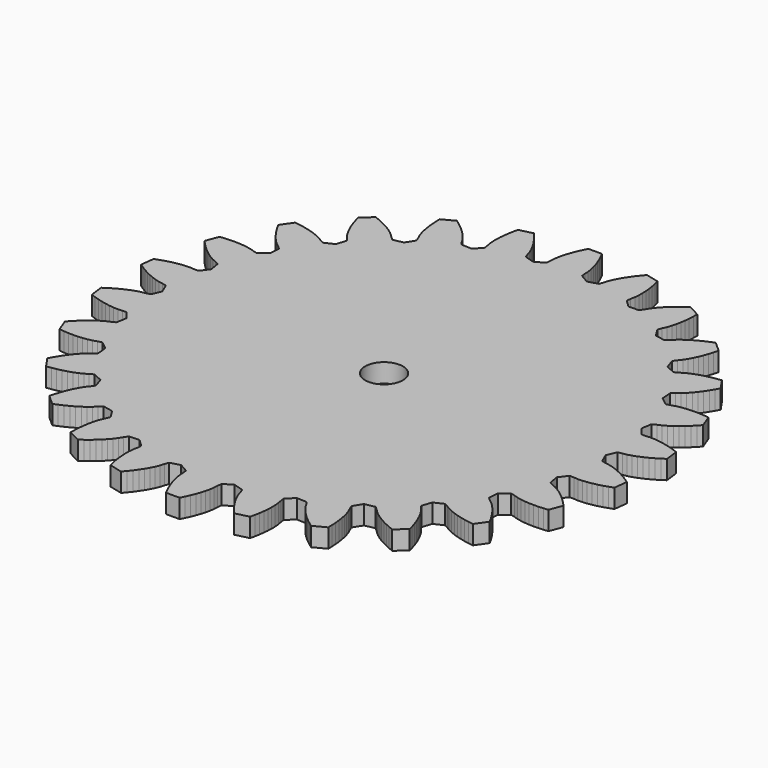
from build123d import *

# Parameters (mm, degrees)
F0_R     = 25.4
F1_DEPTH = 25.4


# Not quite as in the source:
# - ends of sketch curves that miss each other by under 0.0002 mm in the source are joined


with BuildPart() as f1:
    # F0 (on Top) → F1 (new body)
    with BuildSketch(Plane.XY):
        Polygon((93.9964592, 342.9519176), (76.148057, 347.3511722), (71.9280248, 342.4118374), (67.9735496, 337.3908416), (64.2982458, 332.291309), (60.9200458, 327.1156526), (57.8641464, 321.8650154), (55.1692572, 316.5382544), (52.9062696, 311.128791), (51.253517, 305.6119872), (49.2553752, 300.1503776), (35.9741724, 296.2739566), (24.0065814, 303.2161576), (23.3735372, 308.9972484), (23.0890826, 314.7492562), (22.1864174, 320.5430978), (20.8446116, 326.3600026), (19.1340994, 332.1894042), (17.0926506, 338.0231238), (14.744573, 343.854024), (12.1066052, 349.6754754), (9.1912948, 355.4812042), (-9.1912948, 355.4812042), (-12.1066052, 349.6754754), (-14.744573, 343.854024), (-17.0926506, 338.0231238), (-19.1340994, 332.1894042), (-20.8446116, 326.3600026), (-22.1864174, 320.5430978), (-23.0890826, 314.7492562), (-23.3735372, 308.9972484), (-24.0065814, 303.2161576), (-35.9741724, 296.2739566), (-49.2553752, 300.1503776), (-51.253517, 305.6119872), (-52.9062696, 311.128791), (-55.1692572, 316.5382544), (-57.8641464, 321.8650154), (-60.9200458, 327.1156526), (-64.2982458, 332.291309), (-67.9735496, 337.3908416), (-71.9280248, 342.4118374), (-76.1480062, 347.3511722), (-93.9964084, 342.951943), (-95.4376298, 336.6172592), (-96.6057758, 330.3336294), (-97.4902038, 324.1102484), (-98.0762072, 317.9574794), (-98.3419674, 311.888124), (-98.2527118, 305.9191494), (-97.7425782, 300.077632), (-96.6422248, 294.4246842), (-95.8733668, 288.660078), (-105.8318178, 279.0556014), (-119.6548026, 279.6409698), (-122.9019386, 284.4656998), (-125.826901, 289.4266754), (-129.3187152, 294.1373594), (-133.210046, 298.6644014), (-137.4337104, 303.0311694), (-141.9523704, 307.2479504), (-146.741261, 311.3197482), (-151.7824498, 315.2484932), (-157.0618652, 319.0343632), (-173.3388202, 310.4915558), (-173.222158, 303.9960392), (-172.852588, 297.615483), (-172.2219568, 291.3612664), (-171.3185042, 285.2470546), (-170.1240438, 279.2904498), (-168.6089084, 273.5162678), (-166.7156432, 267.9665964), (-164.2944136, 262.7412322), (-162.168332, 257.328162), (-169.5389294, 245.619524), (-183.1003196, 242.8798546), (-187.4077278, 246.787289), (-191.4349232, 250.9040956), (-195.952618, 254.6422644), (-200.8142796, 258.1065196), (-205.9602434, 261.3355708), (-211.3567528, 264.348468), (-216.9809224, 267.1558792), (-222.8158104, 269.7640274), (-228.8478532, 272.1764432), (-242.6074142, 259.9865514), (-240.9396502, 253.7076968), (-239.0538526, 247.600978), (-236.9448144, 241.6793998), (-234.6043822, 235.9590912), (-232.0191448, 230.461439), (-229.166166, 225.2176344), (-225.999802, 220.2823128), (-222.3984122, 215.78824), (-219.038678, 211.041234), (-223.3930254, 197.9089514), (-235.9047098, 192.003426), (-241.0220478, 194.7664888), (-245.917466, 197.7999092), (-251.1984816, 200.3482912), (-256.7479244, 202.5484138), (-262.5171026, 204.4521438), (-268.4778222, 206.0859988), (-274.610449, 207.4658792), (-280.8999462, 208.6018434), (-287.3340456, 209.5006224), (-297.776519, 194.3720522), (-294.654605, 188.6747814), (-291.3621808, 183.1968142), (-287.897316, 177.9520444), (-284.2559212, 172.9580488), (-280.430097, 168.2388304), (-276.4051114, 163.8301778), (-272.1496716, 159.7960228), (-267.5774176, 156.2943788), (-263.1792806, 152.4893826), (-264.2643432, 138.6966238), (-274.9991706, 129.9684726), (-280.6290552, 131.426585), (-286.1081654, 133.2003178), (-291.8455936, 134.4108056), (-297.7602884, 135.2189066), (-303.8174264, 135.686673), (-309.995951, 135.846566), (-316.2805968, 135.7187278), (-322.6591972, 135.3165188), (-329.1214144, 134.6493878), (-335.6399688, 117.4613856), (-331.2453116, 112.6767876), (-326.7375736, 108.1459102), (-322.1182534, 103.8827488), (-317.3875288, 99.905312), (-312.5435202, 96.2387966), (-307.580411, 92.9215058), (-302.4831644, 90.0229594), (-297.2058064, 87.7172998), (-292.0248668, 85.075395), (-289.7775764, 71.4237586), (-298.1116974, 60.3802196), (-303.9269258, 60.4486218), (-309.6713136, 60.8595938), (-315.5317032, 60.6618548), (-321.4679372, 60.030995), (-327.460991, 59.0355944), (-333.4982662, 57.712229), (-339.569679, 56.084089), (-345.6666696, 54.1670494), (-351.7814402, 51.9727942), (-353.9972346, 33.7242658), (-348.5852312, 30.1303944), (-343.1242058, 26.8099794), (-337.618832, 23.7761526), (-332.0737072, 21.04644), (-326.4930224, 18.6457082), (-320.8802574, 16.6125652), (-315.2374696, 15.0181056), (-309.5616618, 14.04239), (-303.8990366, 12.717145), (-298.45, 0), (-303.8990366, -12.7171196), (-309.5616618, -14.0423646), (-315.2374696, -15.0180802), (-320.8802574, -16.6125398), (-326.4930224, -18.6457082), (-332.0737326, -21.0464146), (-337.618832, -23.7761526), (-343.1242058, -26.809954), (-348.5852566, -30.1303944), (-353.9972346, -33.7242404), (-351.7814402, -51.9727942), (-345.6666696, -54.1670494), (-339.569679, -56.0840636), (-333.4982662, -57.7122036), (-327.460991, -59.035569), (-321.4679372, -60.030995), (-315.5317032, -60.6618548), (-309.6713136, -60.8595684), (-303.9269258, -60.4486218), (-298.1116974, -60.3801942), (-289.7775764, -71.4237586), (-292.0248668, -85.0753696), (-297.2058064, -87.7172744), (-302.4831898, -90.022934), (-307.580411, -92.9214804), (-312.5435202, -96.2387712), (-317.3875288, -99.9052866), (-322.1182534, -103.8827234), (-326.737599, -108.1459102), (-331.2453116, -112.6767622), (-335.6399688, -117.4613602), (-329.1214144, -134.6493624), (-322.6591972, -135.3164934), (-316.2805968, -135.7187024), (-309.9959764, -135.8465406), (-303.8174518, -135.6866476), (-297.7603138, -135.2189066), (-291.8455936, -134.4108056), (-286.1081654, -133.2002924), (-280.6290552, -131.4265596), (-274.9991706, -129.9684472), (-264.2643432, -138.6966238), (-263.1792806, -152.4893826), (-267.577443, -156.2943788), (-272.1496716, -159.7959974), (-276.4051368, -163.8301524), (-280.4301224, -168.238805), (-284.2559212, -172.9580234), (-287.897316, -177.952019), (-291.3621808, -183.1967888), (-294.6546304, -188.6747814), (-297.7765444, -194.3720522), (-287.3340456, -209.500597), (-280.8999462, -208.6018434), (-274.610449, -207.4658792), (-268.4778476, -206.0859988), (-262.517128, -204.4521184), (-256.7479244, -202.5483884), (-251.1984816, -200.3482912), (-245.917466, -197.7999092), (-241.0220478, -194.7664888), (-235.9047098, -192.003426), (-223.3930508, -197.9089514), (-219.038678, -211.041234), (-222.3984376, -215.7882146), (-225.999802, -220.2822874), (-229.166166, -225.2176344), (-232.0191448, -230.4614136), (-234.6044076, -235.9590658), (-236.9448398, -241.6793998), (-239.053878, -247.6009526), (-240.9396756, -253.7076968), (-242.6074142, -259.986526), (-228.8478786, -272.1764432), (-222.8158358, -269.764002), (-216.9809478, -267.1558792), (-211.3567528, -264.348468), (-205.9602434, -261.3355708), (-200.814305, -258.1064942), (-195.9526434, -254.6422644), (-191.4349486, -250.9040956), (-187.4077278, -246.7872636), (-183.1003196, -242.8798292), (-169.5389294, -245.619524), (-162.1683574, -257.3281366), (-164.294439, -262.7412322), (-166.7156686, -267.9665964), (-168.6089084, -273.5162678), (-170.1240692, -279.2904498), (-171.3185042, -285.2470292), (-172.2219822, -291.361241), (-172.8526134, -297.6154576), (-173.2221834, -303.9960392), (-173.3388456, -310.4915558), (-157.0618906, -319.0343632), (-151.7824498, -315.2484678), (-146.7412864, -311.3197482), (-141.9523958, -307.2479504), (-137.4337358, -303.031144), (-133.2100714, -298.6644014), (-129.3187152, -294.1373594), (-125.8269264, -289.42665), (-122.9019386, -284.4656744), (-119.654828, -279.6409698), (-105.8318432, -279.0556014), (-95.8733668, -288.660078), (-96.6422502, -294.4246842), (-97.7426036, -300.077632), (-98.2527118, -305.9191494), (-98.3419928, -311.888124), (-98.0762326, -317.9574794), (-97.4902292, -324.110223), (-96.6057758, -330.3336294), (-95.4376298, -336.6172338), (-93.9964338, -342.951943), (-76.1480316, -347.3511722), (-71.9280248, -342.4118374), (-67.9735496, -337.3908416), (-64.2982712, -332.291309), (-60.9200458, -327.1156526), (-57.8641718, -321.8650154), (-55.1692826, -316.5382544), (-52.9062696, -311.128791), (-51.2535424, -305.6119872), (-49.2554006, -300.1503776), (-35.9741978, -296.2739566), (-24.0065814, -303.2161576), (-23.3735626, -308.997223), (-23.089108, -314.7492562), (-22.1864428, -320.5430978), (-20.844637, -326.3600026), (-19.1340994, -332.1894042), (-17.092676, -338.0231238), (-14.744573, -343.854024), (-12.1066052, -349.6754754), (-9.1912948, -355.4812042), (9.1912694, -355.4812042), (12.1065798, -349.6754754), (14.7445476, -343.854024), (17.0926506, -338.0231238), (19.134074, -332.1894042), (20.8446116, -326.3600026), (22.186392, -320.5430978), (23.0890826, -314.7492562), (23.3735372, -308.9972484), (24.006556, -303.2161576), (35.974147, -296.2739566), (49.2553752, -300.1503776), (51.253517, -305.6119872), (52.9062442, -311.1288164), (55.1692572, -316.5382544), (57.864121, -321.8650154), (60.9200204, -327.115678), (64.2982204, -332.2913344), (67.9735242, -337.390867), (71.9279994, -342.4118628), (76.1480062, -347.3511722), (93.9964084, -342.951943), (95.4376044, -336.6172592), (96.6057504, -330.3336548), (97.4901784, -324.1102484), (98.0761818, -317.9575048), (98.3419674, -311.8881494), (98.2526864, -305.9191494), (97.7425782, -300.0776574), (96.6422248, -294.4246842), (95.8733414, -288.6601034), (105.8318178, -279.0556014), (119.6547772, -279.6409952), (122.9019132, -284.4656998), (125.8268756, -289.4266754), (129.3186898, -294.1373594), (133.210046, -298.6644268), (137.433685, -303.0311694), (141.9523704, -307.2479758), (146.741261, -311.3197736), (151.7824244, -315.2484932), (157.0618398, -319.0343886), (173.3388202, -310.4915812), (173.2221326, -303.9960646), (172.852588, -297.615483), (172.2219568, -291.3612664), (171.3184788, -285.2470546), (170.1240438, -279.2904752), (168.608883, -273.5162932), (166.7156432, -267.9665964), (164.2944136, -262.7412576), (162.168332, -257.328162), (169.538904, -245.6195494), (183.1002942, -242.8798546), (187.4077024, -246.787289), (191.4349232, -250.904121), (195.952618, -254.6422898), (200.8142796, -258.1065196), (205.960218, -261.3355962), (211.3567274, -264.348468), (216.980897, -267.1559046), (222.8158104, -269.7640274), (228.8478532, -272.1764686), (242.6073888, -259.9865514), (240.9396248, -253.7077222), (239.0538272, -247.600978), (236.9448144, -241.6794252), (234.6043568, -235.9590912), (232.0191194, -230.461439), (229.1661406, -225.2176598), (225.9997766, -220.2823128), (222.3984122, -215.78824), (219.0386526, -211.0412594), (223.3930254, -197.9089768), (235.9046844, -192.0034514), (241.0220478, -194.7665142), (245.917466, -197.7999346), (251.1984562, -200.3483166), (256.747899, -202.5484138), (262.5171026, -204.4521438), (268.4778222, -206.0860242), (274.6104236, -207.4659046), (280.8999462, -208.6018688), (287.3340202, -209.5006478), (297.776519, -194.3720776), (294.654605, -188.6748068), (291.3621554, -183.1968396), (287.8972906, -177.9520444), (284.2558958, -172.9580488), (280.430097, -168.2388558), (276.4051114, -163.8302032), (272.1496462, -159.7960228), (267.5774176, -156.2944042), (263.1792806, -152.489408), (264.2643432, -138.6966492), (274.9991706, -129.9684726), (280.6290552, -131.426585), (286.1081654, -133.2003178), (291.8455936, -134.410831), (297.7602884, -135.218932), (303.8174264, -135.6866984), (309.995951, -135.8465914), (316.2805968, -135.7187532), (322.6591972, -135.3165188), (329.1214144, -134.6493878), (335.6399688, -117.4613856), (331.2453116, -112.6767876), (326.7375736, -108.1459356), (322.118228, -103.8827488), (317.3875034, -99.905312), (312.5434948, -96.238822), (307.580411, -92.9215058), (302.4831644, -90.0229848), (297.2058064, -87.7172998), (292.0248668, -85.0754204), (289.7775764, -71.423784), (298.111672, -60.3802196), (303.9269258, -60.4486472), (309.6712882, -60.8595938), (315.5317032, -60.6618802), (321.4679372, -60.0310204), (327.460991, -59.0356198), (333.4982408, -57.7122544), (339.569679, -56.0841144), (345.6666696, -54.1670748), (351.7814402, -51.9728196), (353.9972092, -33.7242912), (348.5852312, -30.1304198), (343.1242058, -26.8099794), (337.618832, -23.776178), (332.0737072, -21.0464654), (326.4930224, -18.6457336), (320.8802574, -16.6125652), (315.2374696, -15.0181056), (309.5616618, -14.04239), (303.8990366, -12.717145), (298.45, -2.54e-05), (303.8990366, 12.7170942), (309.5616618, 14.0423392), (315.2374696, 15.0180548), (320.8802574, 16.6125144), (326.4930224, 18.6456828), (332.0737326, 21.0463892), (337.618832, 23.7761272), (343.1242058, 26.8099286), (348.5852566, 30.130369), (353.9972346, 33.724215), (351.7814656, 51.9727688), (345.6666696, 54.167024), (339.569679, 56.0840636), (333.4982662, 57.7121782), (327.4610164, 59.035569), (321.4679372, 60.0309696), (315.5317032, 60.6618294), (309.6713136, 60.859543), (303.9269258, 60.4485964), (298.1116974, 60.3801942), (289.7776018, 71.4237332), (292.0248668, 85.0753696), (297.2058064, 87.717249), (302.4831898, 90.022934), (307.5804364, 92.921455), (312.5435202, 96.2387712), (317.3875288, 99.9052612), (322.1182534, 103.882698), (326.737599, 108.1458848), (331.245337, 112.6767368), (335.6399688, 117.4613348), (329.1214398, 134.649337), (322.6591972, 135.316468), (316.2806222, 135.7187024), (309.9959764, 135.8465406), (303.8174518, 135.6866476), (297.7603138, 135.2188812), (291.8455936, 134.4107802), (286.1081908, 133.200267), (280.6290806, 131.4265596), (274.999196, 129.9684472), (264.2643686, 138.6965984), (263.179306, 152.4893572), (267.577443, 156.2943534), (272.1496716, 159.7959974), (276.4051368, 163.8301524), (280.4301224, 168.238805), (284.2559212, 172.9580234), (287.897316, 177.952019), (291.3622062, 183.1967888), (294.6546304, 188.674756), (297.7765444, 194.3720268), (287.334071, 209.500597), (280.8999716, 208.601818), (274.6104744, 207.4658538), (268.4778476, 206.0859734), (262.517128, 204.4521184), (256.7479498, 202.5483884), (251.198507, 200.3482658), (245.9174914, 197.7998838), (241.0220732, 194.7664634), (235.9047352, 192.0034006), (223.3930508, 197.908926), (219.0387034, 211.0412086), (222.3984376, 215.7882146), (225.9998274, 220.2822874), (229.1661914, 225.217609), (232.0191702, 230.4614136), (234.6044076, 235.9590658), (236.9448398, 241.6793744), (239.053878, 247.6009526), (240.9396756, 253.7076714), (242.6074396, 259.986526), (228.8478786, 272.1764178), (222.8158358, 269.764002), (216.9809478, 267.1558538), (211.3567782, 264.3484426), (205.9602688, 261.3355708), (200.814305, 258.1064942), (195.9526434, 254.6422644), (191.4349486, 250.9040956), (187.4077532, 246.7872636), (183.100345, 242.8798292), (169.5389548, 245.619524), (162.1683574, 257.3281366), (164.294439, 262.7412322), (166.7156686, 267.966571), (168.6089338, 273.5162678), (170.1240692, 279.2904244), (171.3185296, 285.2470292), (172.2220076, 291.361241), (172.8526134, 297.6154576), (173.2221834, 303.9960392), (173.338871, 310.4915558), (157.0618906, 319.0343632), (151.7824752, 315.2484678), (146.7412864, 311.3197482), (141.9524212, 307.2479504), (137.4337358, 303.031144), (133.2100968, 298.6644014), (129.3187406, 294.1373594), (125.8269264, 289.42665), (122.901964, 284.4656744), (119.654828, 279.6409698), (105.8318686, 279.055576), (95.8733922, 288.660078), (96.6422502, 294.4246842), (97.742629, 300.077632), (98.2527372, 305.919124), (98.3420182, 311.888124), (98.0762326, 317.9574794), (97.4902292, 324.110223), (96.6058012, 330.3336294), (95.4376552, 336.6172338), align=None)
        Circle(F0_R, mode=Mode.SUBTRACT)
    extrude(amount=F1_DEPTH)


solid = f1.part
